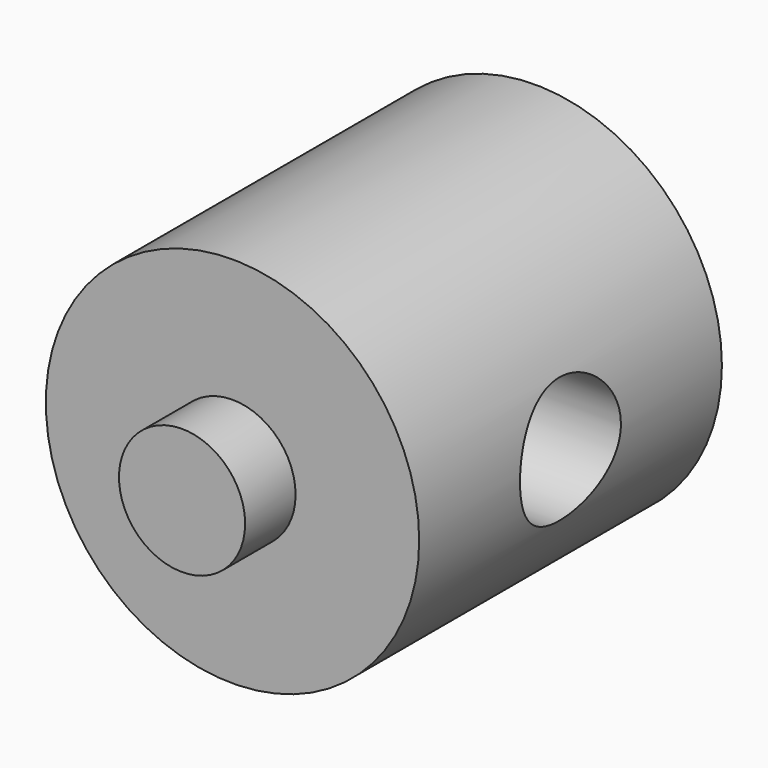
from build123d import *

# Parameters (mm, degrees)
F0_R           = 9.398
F1_DEPTH       = 19.05
F2_R           = 3.175
F3_DEPTH       = 3.175
F4_R           = 3.175
F5_DEPTH       = 3.175
F6_R           = 3.175
F7_DEPTH       = 127
F10_DEPTH      = 25.4
F11_DEPTH      = 25.4
F11_DEPTH_BACK = 25.4


# Not quite as in the source:
# - a feature of the source that left no trace in its solid (it failed there, or was rolled back) is left out


with BuildPart() as f1:
    # F0 (on Front) → F1 (new body)
    with BuildSketch(Plane.XZ):
        Circle(F0_R)
    extrude(amount=F1_DEPTH)

    # F2 (on face) → F3 (join)
    with BuildSketch(Plane.XZ.offset(19.05)):
        Circle(F2_R)
    extrude(amount=F3_DEPTH)

    # F4 (on face) → F5 (join)
    with BuildSketch(Plane(origin=(0, 0, 0), x_dir=(-1, 0, 0), z_dir=(0, 1, 0))):
        Circle(F4_R)
    extrude(amount=F5_DEPTH)

    # F6 (on Right) → F7 (cut)
    with BuildSketch(Plane.YZ):
        with Locations((-9.5303244889, 0)):
            Circle(F6_R)
    extrude(amount=-F7_DEPTH, mode=Mode.SUBTRACT)

    # F6 (on Right) → F10 (cut)
    with BuildSketch(Plane.YZ):
        with Locations((-9.5303244889, 0)):
            Circle(F6_R)
    extrude(amount=-F10_DEPTH, mode=Mode.SUBTRACT)

    # F6 (on Right) → F11 (cut, two sides)
    with BuildSketch(Plane.YZ) as f11_sk:
        with Locations((-9.5303244889, 0)):
            Circle(F6_R)
    extrude(amount=-F11_DEPTH, mode=Mode.SUBTRACT)
    extrude(f11_sk.sketch, amount=F11_DEPTH_BACK, mode=Mode.SUBTRACT)


solid = f1.part
